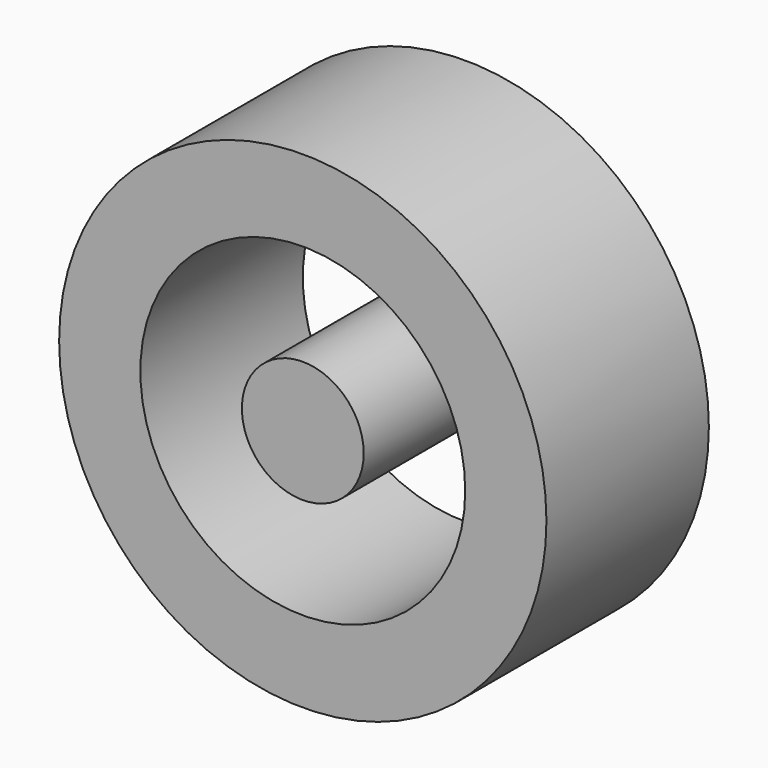
from build123d import *

# Parameters (mm, degrees)
F0_R     = 19.05
F0_R_2   = 12.7
F1_DEPTH = 7.9375
F0_R_3   = 4.7625


# Not quite as in the source:
# - a length typed as a fraction of an inch, garbled in the dataset ("3 / 203.2 mm" for 3/8 in), is restored


with BuildPart() as f1:
    # F0 (on Front) → F1 (new body, symmetric)
    with BuildSketch(Plane.XZ):
        Circle(F0_R)
        Circle(F0_R_2, mode=Mode.SUBTRACT)
    extrude(amount=F1_DEPTH, both=True)


with BuildPart() as f1b:
    # F0 (on Front) → F1, piece 2 (new body, symmetric)
    with BuildSketch(Plane.XZ):
        Circle(F0_R_3)
    extrude(amount=F1_DEPTH, both=True)


solid = Compound([f1.part, f1b.part])
